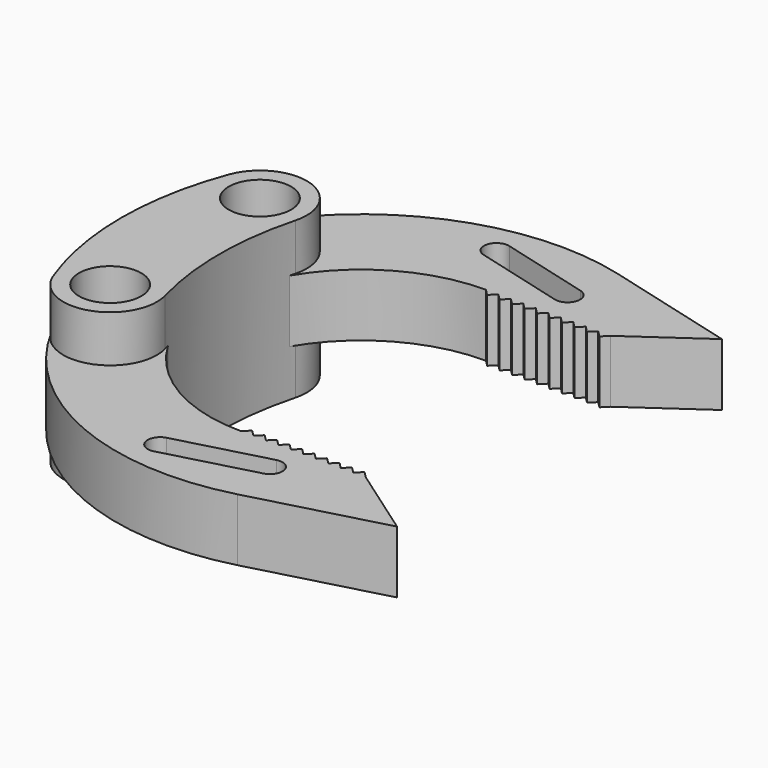
from build123d import *

# Parameters (mm, degrees)
F0_R     = 5
F2_DEPTH = 12.5
F1_R     = 5
F3_DEPTH = 5


# Not quite as in the source:
# - a feature of the source that left no trace in its solid (it failed there, or was rolled back) is left out


with BuildPart() as f2:
    # F0 (on Top) → F2 (new body, symmetric)
    with BuildSketch(Plane.XY):
        with BuildLine():
            ThreePointArc((7.2403054276, -13.0434782609), (5.5090082779, 0), (7.2403054276, 13.0434782609))
            ThreePointArc((7.2403054276, 13.0434782609), (2.3044883911, 22.1371796429), (-7.0173413473, 17.6470588235))
            ThreePointArc((-7.0173413473, 17.6470588235), (-10.2350656985, 0), (-7.0173413473, -17.6470588235))
            ThreePointArc((-7.0173413473, -17.6470588235), (2.3044883911, -22.1371796429), (7.2403054276, -13.0434782609))
        make_face()
        with Locations((0, -15)):
            Circle(F0_R, mode=Mode.SUBTRACT)
        with Locations((0, 15)):
            Circle(F0_R, mode=Mode.SUBTRACT)
    extrude(amount=F2_DEPTH, both=True)

    # F1 (on Top) → F3 (join, symmetric)
    with BuildSketch(Plane.XY):
        with BuildLine():
            ThreePointArc((38.9229935461, 38.1714845638), (12.7620087728, 36.2695311392), (-6.5959822677, 18.5697363943))
            ThreePointArc((-6.5959822677, 18.5697363943), (-3.5697363943, 8.4040177323), (6.5959822677, 11.4302636057))
            ThreePointArc((6.5959822677, 11.4302636057), (15.785676778, 21.0076181762), (28.5825898266, 24.5311422915))
            Line((28.5825898266, 24.5311422915), (30.5825898266, 24.5311422915))
            Line((30.5825898266, 24.5311422915), (32.5825898266, 24.5311422915))
            Line((32.5825898266, 24.5311422915), (34.5825898266, 24.5311422915))
            Line((34.5825898266, 24.5311422915), (36.5825898266, 24.5311422915))
            Line((36.5825898266, 24.5311422915), (38.5825898266, 24.5311422915))
            Line((38.5825898266, 24.5311422915), (40.5825898266, 24.5311422915))
            Line((40.5825898266, 24.5311422915), (42.5825898266, 24.5311422915))
            Line((42.5825898266, 24.5311422915), (44.5825898266, 24.5311422915))
            Line((44.5825898266, 24.5311422915), (46.5825898266, 24.5311422915))
            Line((46.5825898266, 24.5311422915), (48.5825898266, 24.5311422915))
            Line((48.5825898266, 24.5311422915), (60, 32.5311422915))
            Line((60, 32.5311422915), (38.9229935461, 38.1714845638))
        make_face()
        with Locations((0, 15)):
            Circle(F1_R, mode=Mode.SUBTRACT)
        with BuildLine():
            ThreePointArc((22.4425128865, 31.74578129), (21.0275159589, 34.1948185896), (23.4765532585, 35.6098155172))
            Line((23.4765532585, 35.6098155172), (37.9666816106, 31.7321641224))
            ThreePointArc((37.9666816106, 31.7321641224), (39.0361733804, 31.017923595), (39.4496614246, 29.8001470088))
            ThreePointArc((39.4496614246, 29.8001470088), (38.6674380108, 28.2136350529), (36.9326412386, 27.8681298951))
            Line((36.9326412386, 27.8681298951), (22.4425128865, 31.74578129))
        make_face(mode=Mode.SUBTRACT)
        with BuildLine():
            Line((32.5825898266, -24.5311422915), (30.5825898266, -24.5311422915))
            Line((30.5825898266, -24.5311422915), (28.5825898266, -24.5311422915))
            ThreePointArc((28.5825898266, -24.5311422915), (15.785676778, -21.0076181762), (6.5959822677, -11.4302636057))
            ThreePointArc((6.5959822677, -11.4302636057), (-3.5697363943, -8.4040177323), (-6.5959822677, -18.5697363943))
            ThreePointArc((-6.5959822677, -18.5697363943), (12.7620087728, -36.2695311392), (38.9229935461, -38.1714845638))
            Line((38.9229935461, -38.1714845638), (60, -32.5311422915))
            Line((60, -32.5311422915), (48.5825898266, -24.5311422915))
            Line((48.5825898266, -24.5311422915), (46.5825898266, -24.5311422915))
            Line((46.5825898266, -24.5311422915), (44.5825898266, -24.5311422915))
            Line((44.5825898266, -24.5311422915), (42.5825898266, -24.5311422915))
            Line((42.5825898266, -24.5311422915), (40.5825898266, -24.5311422915))
            Line((40.5825898266, -24.5311422915), (38.5825898266, -24.5311422915))
            Line((38.5825898266, -24.5311422915), (36.5825898266, -24.5311422915))
            Line((36.5825898266, -24.5311422915), (34.5825898266, -24.5311422915))
            Line((34.5825898266, -24.5311422915), (32.5825898266, -24.5311422915))
        make_face()
        with Locations((0, -15)):
            Circle(F1_R, mode=Mode.SUBTRACT)
        with BuildLine():
            ThreePointArc((23.4765532585, -35.6098155172), (21.0275159589, -34.1948185896), (22.4425128865, -31.74578129))
            Line((22.4425128865, -31.74578129), (36.9326412386, -27.8681298951))
            ThreePointArc((36.9326412386, -27.8681298951), (38.6674380108, -28.2136350529), (39.4496614246, -29.8001470088))
            ThreePointArc((39.4496614246, -29.8001470088), (39.0361733804, -31.017923595), (37.9666816106, -31.7321641224))
            Line((37.9666816106, -31.7321641224), (23.4765532585, -35.6098155172))
        make_face(mode=Mode.SUBTRACT)
        Polygon((30.5825898266, 24.5311422915), (28.5825898266, 24.5311422915), (29.5825898266, 23.5311422915), align=None)
        Polygon((32.5825898266, 24.5311422915), (30.5825898266, 24.5311422915), (31.5825898266, 23.5311422915), align=None)
        Polygon((34.5825898266, 24.5311422915), (32.5825898266, 24.5311422915), (33.5825898266, 23.5311422915), align=None)
        Polygon((36.5825898266, 24.5311422915), (34.5825898266, 24.5311422915), (35.5825898266, 23.5311422915), align=None)
        Polygon((38.5825898266, 24.5311422915), (36.5825898266, 24.5311422915), (37.5825898266, 23.5311422915), align=None)
        Polygon((40.5825898266, 24.5311422915), (38.5825898266, 24.5311422915), (39.5825898266, 23.5311422915), align=None)
        Polygon((41.5825898266, 23.5311422915), (42.5825898266, 24.5311422915), (40.5825898266, 24.5311422915), align=None)
        Polygon((43.5825898266, 23.5311422915), (44.5825898266, 24.5311422915), (42.5825898266, 24.5311422915), align=None)
        Polygon((45.5825898266, 23.5311422915), (46.5825898266, 24.5311422915), (44.5825898266, 24.5311422915), align=None)
        Polygon((47.5825898266, 23.5311422915), (48.5825898266, 24.5311422915), (46.5825898266, 24.5311422915), align=None)
        Polygon((30.5825898266, -24.5311422915), (29.5825898266, -23.5311422915), (28.5825898266, -24.5311422915), align=None)
        Polygon((31.5825898266, -23.5311422915), (30.5825898266, -24.5311422915), (32.5825898266, -24.5311422915), align=None)
        Polygon((33.5825898266, -23.5311422915), (32.5825898266, -24.5311422915), (34.5825898266, -24.5311422915), align=None)
        Polygon((35.5825898266, -23.5311422915), (34.5825898266, -24.5311422915), (36.5825898266, -24.5311422915), align=None)
        Polygon((37.5825898266, -23.5311422915), (36.5825898266, -24.5311422915), (38.5825898266, -24.5311422915), align=None)
        Polygon((39.5825898266, -23.5311422915), (38.5825898266, -24.5311422915), (40.5825898266, -24.5311422915), align=None)
        Polygon((41.5825898266, -23.5311422915), (40.5825898266, -24.5311422915), (42.5825898266, -24.5311422915), align=None)
        Polygon((43.5825898266, -23.5311422915), (42.5825898266, -24.5311422915), (44.5825898266, -24.5311422915), align=None)
        Polygon((44.5825898266, -24.5311422915), (46.5825898266, -24.5311422915), (45.5825898266, -23.5311422915), align=None)
        Polygon((46.5825898266, -24.5311422915), (48.5825898266, -24.5311422915), (47.5825898266, -23.5311422915), align=None)
    extrude(amount=F3_DEPTH, both=True)


solid = f2.part
